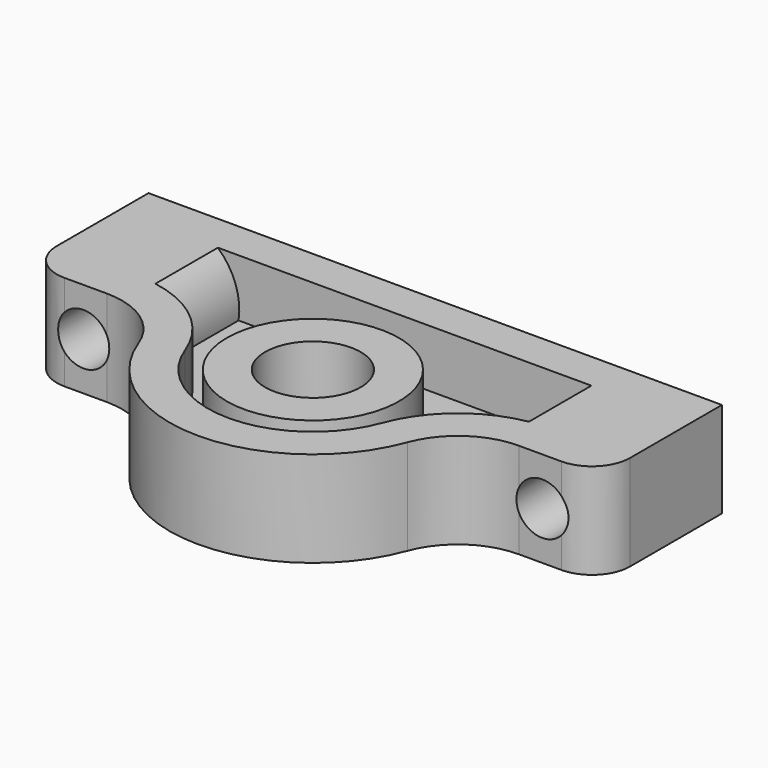
from build123d import *

# Parameters (mm, degrees)
F1_DEPTH    = 6.35
F2_R        = 5.08
F3_R        = 1.7145
F5_DEPTH    = 19.686
F6_T        = 2.54
F7_T1_DEPTH = 19.05


# Not quite as in the source:
# - a fillet or chamfer that OpenCascade refuses, or shapes differently, is made with other operations: its cross-section is extruded or revolved along the edge and cut away or added
# - a shell that OpenCascade refuses in one call is made with other operations: the cavity is built on its own and cut out
# - a feature names something its author has since deleted; it is built from what else it names


with BuildPart() as f1:
    # F0 (on Top) → F1 (new body)
    with BuildSketch(Plane.XY):
        with BuildLine():
            Line((9.525, 0), (3.175, 0))
            ThreePointArc((3.175, 0), (0, -3.175), (-3.175, 0))
            Line((-3.175, 0), (-9.525, 0))
            ThreePointArc((-9.525, 0), (0, -9.525), (9.525, 0))
        make_face()
        with BuildLine():
            ThreePointArc((-3.175, 0), (0, 3.175), (3.175, 0))
            Line((3.175, 0), (9.525, 0))
            ThreePointArc((9.525, 0), (0, 9.525), (-9.525, 0))
            Line((-9.525, 0), (-3.175, 0))
        make_face()
        with BuildLine():
            ThreePointArc((-9.525, 0), (0, 9.525), (9.525, 0))
            Line((9.525, 0), (19.05, 0))
            Line((19.05, 0), (19.05, 10.16))
            Line((19.05, 10.16), (-19.05, 10.16))
            Line((-19.05, 10.16), (-19.05, 0))
            Line((-19.05, 0), (-9.525, 0))
        make_face()
    extrude(amount=F1_DEPTH)

    # F2
    f2_edges = [f1.edges().sort_by_distance(p)[0] for p in [
        (9.525, 0, 3.175),
        (-9.525, 0, 3.175),
    ]]
    fillet(f2_edges, radius=F2_R)

    # F3 (on face) → F5 (cut, through all)
    with BuildSketch(Plane(origin=(0, 10.16, 0), x_dir=(-1, 0, 0), z_dir=(0, 1, 0))):
        with Locations((15.24, 3.175)):
            Circle(F3_R)
        with Locations((-15.24, 3.175)):
            Circle(F3_R)
    extrude(amount=-F5_DEPTH, mode=Mode.SUBTRACT)

    # F6: shell of thickness 2.54, made by hand


with BuildPart() as f6_core1:
    # F6_t2: copy of F1
    add(f1.part)

    # the walls: a layer under each face that stays
    f6_faces = [f6_core1.faces().sort_by_distance(p)[0] for p in [
        (0, -9.525, 3.175),
        (-12.7, 0.3175, 0),
        (-10.7921658217, -0.9097158891, 3.175),
        (10.7921658217, -0.9097158891, 3.175),
        (-18.1571750408, 0, 5.2916666667),
        (14.5858752038, 0, 5.2916666667),
        (-19.05, 5.08, 3.175),
        (19.05, 5.08, 3.175),
        (0, 10.16, 3.175),
        (3.175, 0, 3.175),
        (-13.5255, 5.0786180746, 3.175),
        (16.9545, 5.0786180746, 3.175),
    ]]
    thicken(f6_faces, amount=-F6_T, mode=Mode.SUBTRACT)


with BuildPart() as f1_1:
    add(f1.part)

    # what is left inside the walls is the cavity
    f6_cavity = [f6_core1.part.solids().sort_by_distance(p)[0] for p in [
        (-6.204007, 2.751667, 6.3246),
    ]]
    add(f6_cavity, mode=Mode.SUBTRACT)

    # F7: fillet of radius 2.54 on 2 edges, made by hand

    # F7_s2 → F7_t1 (cut)
    with BuildSketch(Plane.XY.offset(-6.35)):
        with BuildLine():
            ThreePointArc((-16.51, 0), (-18.3060512242, 0.7439487758), (-19.05, 2.54))
            Line((-19.05, 2.54), (-19.05, 0))
            Line((-19.05, 0), (-16.51, 0))
        make_face()
        with BuildLine():
            ThreePointArc((16.51, 0), (18.3060512242, 0.7439487758), (19.05, 2.54))
            Line((19.05, 2.54), (19.05, 0))
            Line((19.05, 0), (16.51, 0))
        make_face()
    extrude(amount=F7_T1_DEPTH, mode=Mode.SUBTRACT)


solid = f1_1.part
